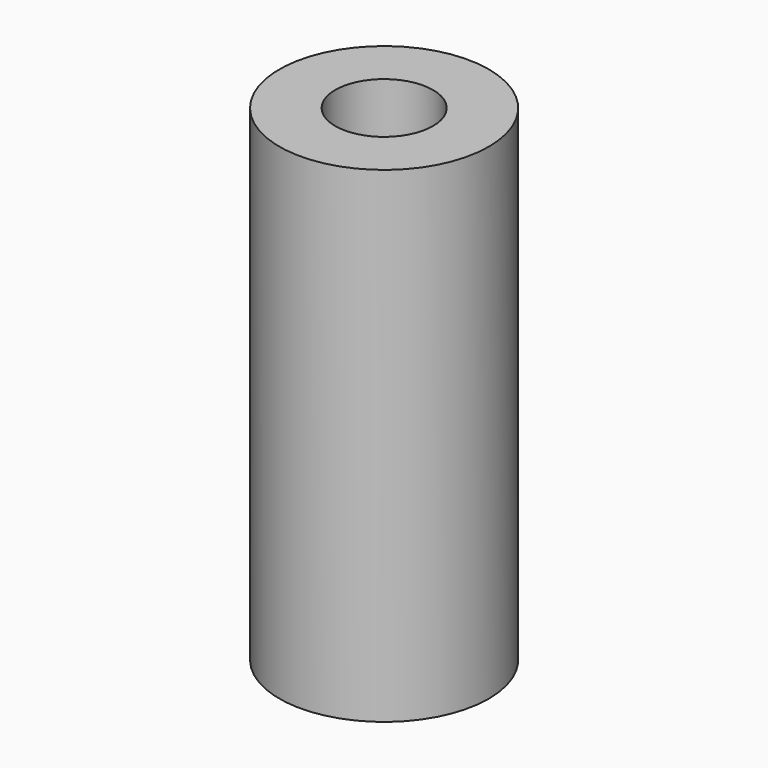
from build123d import *

# Parameters (mm, degrees)
F0_R     = 27.3699899023
F0_R_2   = 12.7730853856
F2_DEPTH = 127


# Not quite as in the source:
# - the program builds the solid bodies; features that only make, move or delete a surface that nothing else refers to are left out


with BuildPart() as f2:
    # F0 (on Top) → F2 (new body)
    with BuildSketch(Plane.XY):
        Circle(F0_R)
        Circle(F0_R_2, mode=Mode.SUBTRACT)
    extrude(amount=F2_DEPTH)


solid = f2.part
